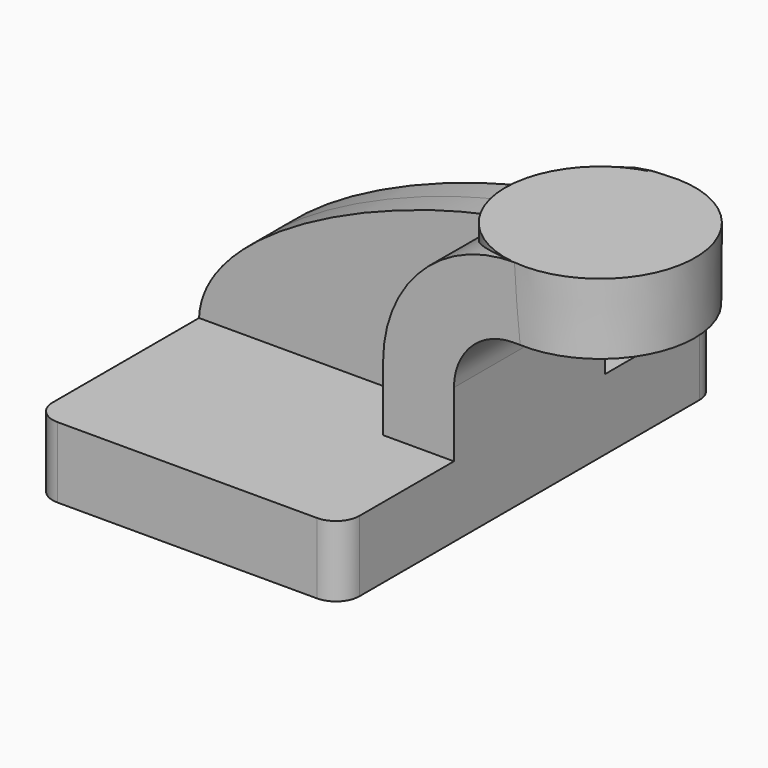
from build123d import *

# Parameters (mm, degrees)
F1_DEPTH = 63.5
F2_DEPTH = 25.4
F3_DEPTH = 7.9375
F4_R     = 6.35


with BuildPart() as f1:
    # F0 (on Front) → F1 (new body, symmetric)
    with BuildSketch(Plane.XZ):
        Polygon((-41.275, -9.525), (41.275, -9.525), (41.275, 9.525), (22.225, 9.525), (-41.275, 9.525), align=None)
    extrude(amount=F1_DEPTH, both=True)

    # F0 (on Front) → F2 (join, symmetric)
    with BuildSketch(Plane.XZ):
        with BuildLine():
            Line((22.225, 9.525), (41.275, 9.525))
            Line((41.275, 9.525), (41.275, 27.0002))
            ThreePointArc((41.275, 27.0002), (45.9246798487, 38.2255201513), (57.15, 42.8752))
            Line((57.15, 42.8752), (60.325, 42.8752))
            Line((60.325, 42.8752), (60.325, 61.9252))
            Line((60.325, 61.9252), (57.15, 61.9252))
            add(Edge.make_bspline(
                [(53.8173720822, 61.7658326875), (54.9505591394, 61.8408261866), (56.0622461787, 61.8941638054), (57.15, 61.9252)],
                knots=[108.1113735744, 108.1113735744, 108.1113735744, 108.1113735744, 111.5045361635, 111.5045361635, 111.5045361635, 111.5045361635], degree=3))
            ThreePointArc((53.8173720822, 61.7658326875), (31.3028758367, 50.4881074735), (22.225, 27.0002))
            Line((22.225, 27.0002), (22.225, 9.525))
        make_face()
    extrude(amount=F2_DEPTH, both=True)

    # F0 (on Front) → F3 (join, symmetric)
    with BuildSketch(Plane.XZ):
        with BuildLine():
            add(Edge.make_bspline(
                [(-41.275, 9.525), (-40.218694031, 35.0028870222), (17.7122913335, 59.3764245807), (53.8173720822, 61.7658326875)],
                knots=[0, 0, 0, 0, 108.1113735744, 108.1113735744, 108.1113735744, 108.1113735744], degree=3))
            Line((-41.275, 9.525), (22.225, 9.525))
            Line((22.225, 9.525), (22.225, 27.0002))
            ThreePointArc((22.225, 27.0002), (31.3028758367, 50.4881074735), (53.8173720822, 61.7658326875))
        make_face()
    extrude(amount=F3_DEPTH, both=True)

    # F4
    f4_edges = [f1.edges().sort_by_distance(p)[0] for p in [
        (-41.275, -63.5, 0),
        (41.275, -63.5, 0),
        (41.275, 63.5, 0),
        (-41.275, 63.5, 0),
    ]]
    fillet(f4_edges, radius=F4_R)

    # F0 (on Front) → F5 (revolve)
    with BuildSketch(Plane.XZ):
        Polygon((60.325, 61.9252), (60.325, 42.8752), (85.7551261626, 42.8752), (85.8753103219, 61.9252), align=None)
    revolve(axis=Axis((60.325, 0, 52.3875), (0, 0, 1)))


solid = f1.part
